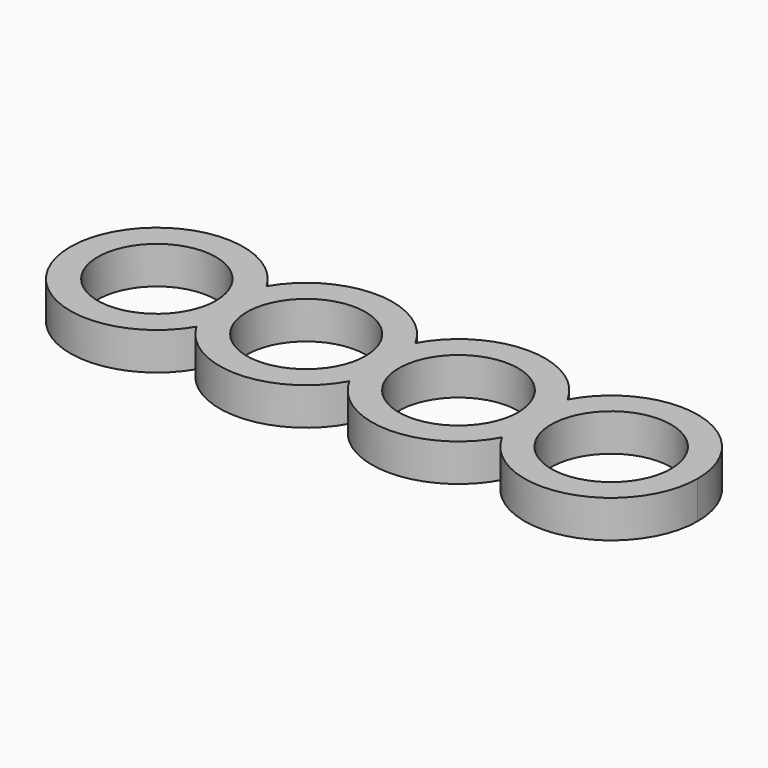
from build123d import *

# Parameters (mm, degrees)
F1_DEPTH = 7


with BuildPart() as f1:
    # F0 (on Top) → F1 (new body)
    with BuildSketch(Plane.XY):
        with BuildLine():
            Line((-31.3795059258, 0), (-26.922398242, 0))
            ThreePointArc((-26.922398242, 0), (-27.4894668745, 4.2460498939), (-29.1509244493, 8.1944755629))
            ThreePointArc((-29.1509244493, 8.1944755629), (-30.8124227539, 4.246057146), (-31.3795059258, 0))
        make_face()
        with BuildLine():
            Line((-26.2997059258, 0), (-26.922398242, 0))
            ThreePointArc((-26.922398242, 0), (-27.4894668745, -4.2460498939), (-29.1509244493, -8.1944755629))
            ThreePointArc((-29.1509244493, -8.1944755629), (-14.9190087878, -16.1773649633), (-0.9726024938, -7.7055470911))
            ThreePointArc((-0.9726024938, -7.7055470911), (-2.4295294135, -3.9745590906), (-2.9252990617, 0))
            Line((-2.9252990617, 0), (-4.0997059258, 0))
            ThreePointArc((-4.0997059258, 0), (-15.1997059258, -11.1), (-26.2997059258, 0))
        make_face()
        with BuildLine():
            ThreePointArc((-29.1509244493, 8.1944755629), (-27.4894668745, 4.2460498939), (-26.922398242, 0))
            Line((-26.922398242, 0), (-26.2997059258, 0))
            ThreePointArc((-26.2997059258, 0), (-15.1997059258, 11.1), (-4.0997059258, 0))
            Line((-4.0997059258, 0), (-2.9252990617, 0))
            ThreePointArc((-2.9252990617, 0), (-2.4295294135, 3.9745590906), (-0.9726024938, 7.7055470911))
            ThreePointArc((-0.9726024938, 7.7055470911), (-14.9190087878, 16.1773649633), (-29.1509244493, 8.1944755629))
        make_face()
        with BuildLine():
            ThreePointArc((-29.1509244493, -8.1944755629), (-27.4894668745, -4.2460498939), (-26.922398242, 0))
            Line((-26.922398242, 0), (-31.3795059258, 0))
            ThreePointArc((-31.3795059258, 0), (-30.8124227539, -4.246057146), (-29.1509244493, -8.1944755629))
        make_face()
        with BuildLine():
            ThreePointArc((-31.3795059258, 0), (-30.8124227539, 4.246057146), (-29.1509244493, 8.1944755629))
            ThreePointArc((-29.1509244493, 8.1944755629), (-47.3485941376, 15.6130773691), (-59.2826902453, 0))
            Line((-59.2826902453, 0), (-54.1525442436, 0))
            ThreePointArc((-54.1525442436, 0), (-43.1025442436, 11.05), (-32.0525442436, 0))
            Line((-32.0525442436, 0), (-31.3795059258, 0))
        make_face()
        with BuildLine():
            ThreePointArc((-59.2826902453, 0), (-47.3485941376, -15.6130773691), (-29.1509244493, -8.1944755629))
            ThreePointArc((-29.1509244493, -8.1944755629), (-30.8124227539, -4.246057146), (-31.3795059258, 0))
            Line((-31.3795059258, 0), (-32.0525442436, 0))
            ThreePointArc((-32.0525442436, 0), (-43.1025442436, -11.05), (-54.1525442436, 0))
            Line((-54.1525442436, 0), (-59.2826902453, 0))
        make_face()
        with BuildLine():
            ThreePointArc((27.5160949741, 7.6415223351), (13.2908629072, 16.1797591406), (-0.9726024938, 7.7055470911))
            ThreePointArc((-0.9726024938, 7.7055470911), (0.4843244259, 3.9745590906), (0.9800940742, 0))
            Line((0.9800940742, 0), (2.1045009383, 0))
            ThreePointArc((2.1045009383, 0), (13.2545009383, 11.15), (24.4045009383, 0))
            Line((24.4045009383, 0), (25.5978890099, 0))
            ThreePointArc((25.5978890099, 0), (26.0847659676, 3.9393012616), (27.5160949741, 7.6415223351))
        make_face()
        with BuildLine():
            ThreePointArc((0.9800940742, 0), (0.4843244259, 3.9745590906), (-0.9726024938, 7.7055470911))
            ThreePointArc((-0.9726024938, 7.7055470911), (-2.4295294135, 3.9745590906), (-2.9252990617, 0))
            Line((-2.9252990617, 0), (0, 0))
            Line((0, 0), (0.9800940742, 0))
        make_face()
        with BuildLine():
            ThreePointArc((-2.9252990617, 0), (-2.4295294135, -3.9745590906), (-0.9726024938, -7.7055470911))
            ThreePointArc((-0.9726024938, -7.7055470911), (0.4843244259, -3.9745590906), (0.9800940742, 0))
            Line((0.9800940742, 0), (0, 0))
            Line((0, 0), (-2.9252990617, 0))
        make_face()
        with BuildLine():
            ThreePointArc((0.9800940742, 0), (0.4843244259, -3.9745590906), (-0.9726024938, -7.7055470911))
            ThreePointArc((-0.9726024938, -7.7055470911), (13.2908629072, -16.1797591406), (27.5160949741, -7.6415223351))
            ThreePointArc((27.5160949741, -7.6415223351), (26.0847659676, -3.9393012616), (25.5978890099, 0))
            Line((25.5978890099, 0), (24.4045009383, 0))
            ThreePointArc((24.4045009383, 0), (13.2545009383, -11.15), (2.1045009383, 0))
            Line((2.1045009383, 0), (0.9800940742, 0))
        make_face()
        with BuildLine():
            ThreePointArc((57.9574890099, 0), (45.7169902715, 15.6929230423), (27.5160949741, 7.6415223351))
            ThreePointArc((27.5160949741, 7.6415223351), (28.9474239806, 3.9393012616), (29.4343009383, 0))
            Line((29.4343009383, 0), (30.5776890099, 0))
            ThreePointArc((30.5776890099, 0), (41.7776890099, 11.2), (52.9776890099, 0))
            Line((52.9776890099, 0), (57.9574890099, 0))
        make_face()
        with BuildLine():
            ThreePointArc((29.4343009383, 0), (28.9474239806, 3.9393012616), (27.5160949741, 7.6415223351))
            ThreePointArc((27.5160949741, 7.6415223351), (26.0847659676, 3.9393012616), (25.5978890099, 0))
            Line((25.5978890099, 0), (29.4343009383, 0))
        make_face()
        with BuildLine():
            ThreePointArc((25.5978890099, 0), (26.0847659676, -3.9393012616), (27.5160949741, -7.6415223351))
            ThreePointArc((27.5160949741, -7.6415223351), (28.9474239806, -3.9393012616), (29.4343009383, 0))
            Line((29.4343009383, 0), (25.5978890099, 0))
        make_face()
        with BuildLine():
            ThreePointArc((29.4343009383, 0), (28.9474239806, -3.9393012616), (27.5160949741, -7.6415223351))
            ThreePointArc((27.5160949741, -7.6415223351), (45.7169902715, -15.6929230423), (57.9574890099, 0))
            Line((57.9574890099, 0), (52.9776890099, 0))
            ThreePointArc((52.9776890099, 0), (41.7776890099, -11.2), (30.5776890099, 0))
            Line((30.5776890099, 0), (29.4343009383, 0))
        make_face()
    extrude(amount=F1_DEPTH)


solid = f1.part
